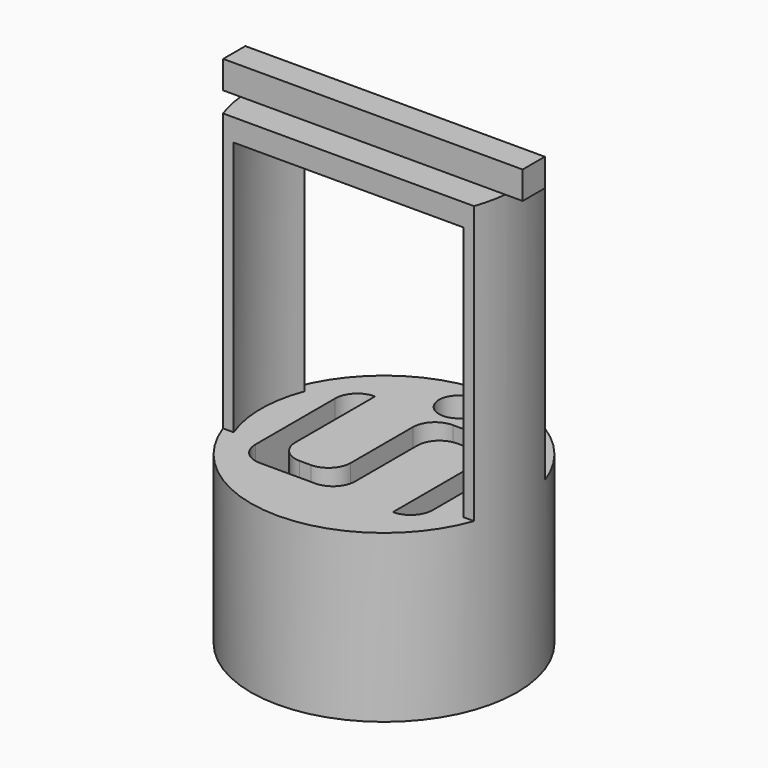
from build123d import *

# Parameters (mm, degrees)
F0_R      = 12
F1_DEPTH  = 15
F2_W      = 2
F2_H      = 2
F2_W_2    = 5
F2_H_2    = 9
F2_H_3    = 11
F3_DEPTH  = 13
F4_R      = 12
F4_R_2    = 11.1
F5_DEPTH  = 25
F7_DEPTH  = 25
F8_W      = 22.627416998
F8_H      = 8
F9_DEPTH  = 2
F10_W     = 27
F10_H     = 2.5
F11_DEPTH = 2.5
F12_R     = 2
F13_R     = 1.99999
F14_R     = 1.75
F15_DEPTH = 13


# Not quite as in the source:
# - a fillet or chamfer is up to 0.001 mm smaller than in the source, because OpenCascade refuses the exact size


with BuildPart() as f1:
    # F0 (on Top) → F1 (new body)
    with BuildSketch(Plane.XY):
        Circle(F0_R)
    extrude(amount=F1_DEPTH)

    # F2 (on face) → F3 (cut)
    with BuildSketch(Plane.XY.offset(15)):
        with Locations((0, 5.5)):
            Rectangle(F2_W, F2_H)
        with Locations((3.5, 5.5)):
            Rectangle(F2_W_2, F2_H)
        Rectangle(F2_W, F2_H_2)
        with Locations((7, 5.5)):
            Rectangle(F2_W, F2_H)
        with Locations((0, -5.5)):
            Rectangle(F2_W, F2_H)
        with Locations((7, -1)):
            Rectangle(F2_W, F2_H_3)
        with Locations((-3.5, -5.5)):
            Rectangle(F2_W_2, F2_H)
        with Locations((-7, -5.5)):
            Rectangle(F2_W, F2_H)
        with Locations((-7, 1)):
            Rectangle(F2_W, F2_H_3)
    extrude(amount=-F3_DEPTH, mode=Mode.SUBTRACT)

    # F4 (on face) → F5 (join)
    with BuildSketch(Plane.XY.offset(15)):
        Circle(F4_R)
        Circle(F4_R_2, mode=Mode.SUBTRACT)
    extrude(amount=F5_DEPTH)

    # F6 (on face) → F7 (cut)
    with BuildSketch(Plane.XY.offset(40)):
        with BuildLine():
            Line((14.9746745975, -4), (14.8116537966, -4))
            Line((14.8116537966, -4), (11.313708499, -4))
            ThreePointArc((11.313708499, -4), (0, -12), (-11.313708499, -4))
            Line((-11.313708499, -4), (-14.8116537966, -4))
            Line((-14.8116537966, -4), (-14.8116537966, -14.8480758196))
            Line((-14.8116537966, -14.8480758196), (14.9746745975, -14.8480758196))
            Line((14.9746745975, -14.8480758196), (14.9746745975, -4))
        make_face()
        with BuildLine():
            Line((11.313708499, -4), (14.8116537966, -4))
            Line((14.8116537966, -4), (14.8116537966, 4))
            Line((14.8116537966, 4), (11.313708499, 4))
            ThreePointArc((11.313708499, 4), (11.8271827158, 2.0292237447), (12, 0))
            ThreePointArc((12, 0), (11.8271827158, -2.0292237447), (11.313708499, -4))
        make_face()
        with BuildLine():
            ThreePointArc((-11.313708499, -4), (0, -12), (11.313708499, -4))
            Line((11.313708499, -4), (10.3542261903, -4))
            ThreePointArc((10.3542261903, -4), (0, -11.1), (-10.3542261903, -4))
            Line((-10.3542261903, -4), (-11.313708499, -4))
        make_face()
        with BuildLine():
            Line((11.313708499, 4), (14.8116537966, 4))
            Line((14.8116537966, 4), (15.4569065875, 4))
            Line((15.4569065875, 4), (15.4569065875, 13.0318450025))
            Line((15.4569065875, 13.0318450025), (-14.8116537966, 13.0318450025))
            Line((-14.8116537966, 13.0318450025), (-14.8116537966, 4))
            Line((-14.8116537966, 4), (-11.313708499, 4))
            ThreePointArc((-11.313708499, 4), (0, 12), (11.313708499, 4))
        make_face()
        with BuildLine():
            Line((-10.3542261903, -4), (10.3542261903, -4))
            ThreePointArc((10.3542261903, -4), (10.9119638634, -2.0344642154), (11.1, 0))
            ThreePointArc((11.1, 0), (10.9119638634, 2.0344642154), (10.3542261903, 4))
            Line((10.3542261903, 4), (-10.3542261903, 4))
            ThreePointArc((-10.3542261903, 4), (-11.1, 0), (-10.3542261903, -4))
        make_face()
        with BuildLine():
            Line((10.3542261903, 4), (11.313708499, 4))
            ThreePointArc((11.313708499, 4), (0, 12), (-11.313708499, 4))
            Line((-11.313708499, 4), (-10.3542261903, 4))
            ThreePointArc((-10.3542261903, 4), (0, 11.1), (10.3542261903, 4))
        make_face()
    extrude(amount=-F7_DEPTH, mode=Mode.SUBTRACT)

    # F8 (on face) → F9 (join)
    with BuildSketch(Plane.XY.offset(40)):
        Rectangle(F8_W, F8_H)
    extrude(amount=-F9_DEPTH)

    # F10 (on face) → F11 (join)
    with BuildSketch(Plane.XY.offset(40)):
        Rectangle(F10_W, F10_H)
    extrude(amount=F11_DEPTH)

    # F12
    f12_edges = [f1.edges().sort_by_distance(p)[0] for p in [
        (-1, -4.5, 8.5),
        (-6, -4.5, 8.5),
        (6, 4.5, 8.5),
        (1, 4.5, 8.5),
    ]]
    fillet(f12_edges, radius=F12_R)

    # F13 (radius 2 in the source; OpenCascade refuses exactly that, so slightly less here)
    f13_edges = [f1.edges().sort_by_distance(p)[0] for p in [
        (-8, 6.5, 8.5),
        (-1, 6.5, 8.5),
        (8, 6.5, 8.5),
        (-8, -6.5, 8.5),
        (1, -6.5, 8.5),
        (8, -6.5, 8.5),
    ]]
    fillet(f13_edges, radius=F13_R)

    # F14 (on face) → F15 (cut)
    with BuildSketch(Plane.XY.offset(15)):
        with Locations((-0.4142135624, 8.9106783271)):
            Circle(F14_R)
    extrude(amount=-F15_DEPTH, mode=Mode.SUBTRACT)


solid = f1.part
